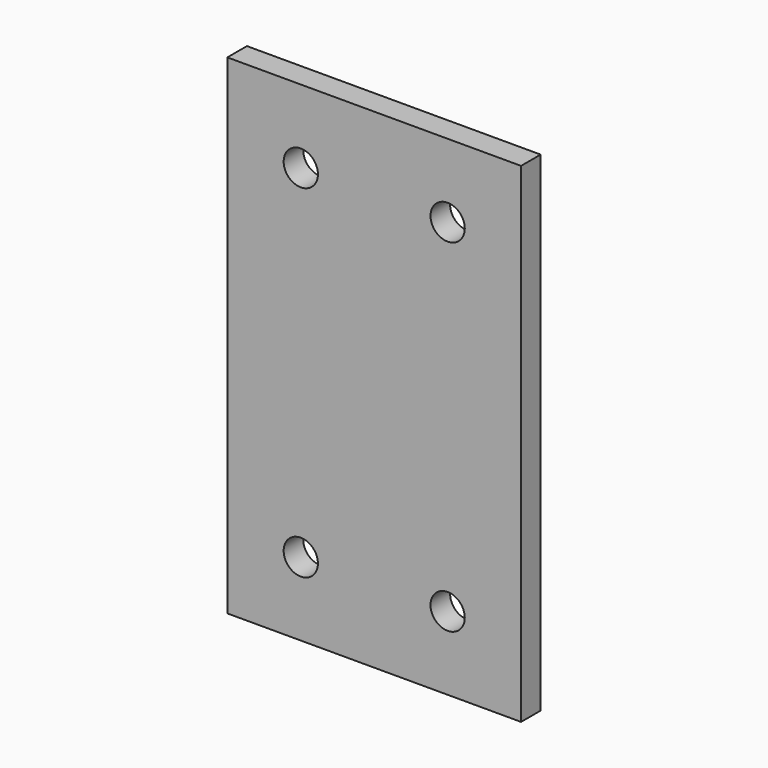
from build123d import *

# Parameters (mm, degrees)
F0_W     = 120
F0_H     = 200
F0_R     = 7
F1_DEPTH = 10


# Not quite as in the source:
# - a feature names something its author has since deleted; it is built from what else it names


with BuildPart() as f1:
    # F0 (on Front) → F1 (new body)
    with BuildSketch(Plane.XZ):
        Rectangle(F0_W, F0_H)
        with Locations((-30, -70)):
            Circle(F0_R, mode=Mode.SUBTRACT)
        with Locations((30, -70)):
            Circle(F0_R, mode=Mode.SUBTRACT)
        with Locations((-30, 70)):
            Circle(F0_R, mode=Mode.SUBTRACT)
        with Locations((30, 70)):
            Circle(F0_R, mode=Mode.SUBTRACT)
    extrude(amount=F1_DEPTH)


solid = f1.part
